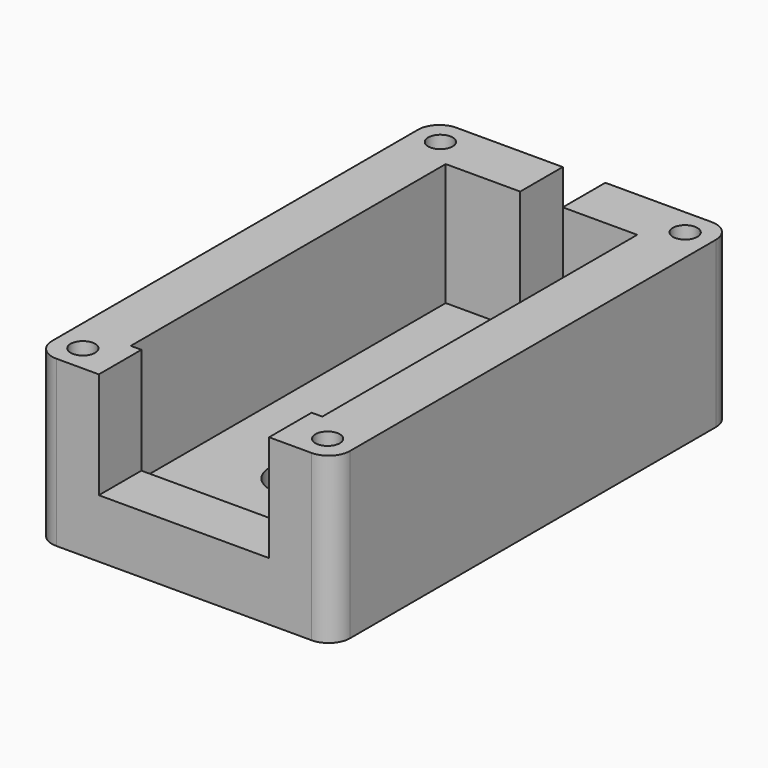
from build123d import *

# Parameters (mm, degrees)
F0_W           = 28
F0_H           = 47
F0_R           = 1.15
F0_W_2         = 18
F0_H_2         = 37
F1_DEPTH       = 11.5
F2_W           = 28
F2_H           = 47
F2_R           = 1.15
F2_W_2         = 18
F2_H_2         = 37
F3_DEPTH       = 4
F4_W           = 16
F4_H           = 5
F4_W_2         = 4
F5_DEPTH       = 10
F6_R           = 2
F8_D           = 2.9
F8_CBORE_D     = 5.5
F8_CBORE_DEPTH = 2.5


with BuildPart() as f1:
    # F0 (on Top) → F1 (new body)
    with BuildSketch(Plane.XY):
        Rectangle(F0_W, F0_H)
        with Locations((-11.5, -21)):
            Circle(F0_R, mode=Mode.SUBTRACT)
        with Locations((11.5, -21)):
            Circle(F0_R, mode=Mode.SUBTRACT)
        with Locations((-11.5, 21)):
            Circle(F0_R, mode=Mode.SUBTRACT)
        Rectangle(F0_W_2, F0_H_2, mode=Mode.SUBTRACT)
        with Locations((11.5, 21)):
            Circle(F0_R, mode=Mode.SUBTRACT)
    extrude(amount=F1_DEPTH)

    # F2 (on face) → F3 (join)
    with BuildSketch(Plane(origin=(0, 0, 0), x_dir=(1, 0, 0), z_dir=(0, 0, -1))):
        Rectangle(F2_W, F2_H)
        with Locations((-11.5, -21)):
            Circle(F2_R, mode=Mode.SUBTRACT)
        with Locations((11.5, -21)):
            Circle(F2_R, mode=Mode.SUBTRACT)
        with Locations((-11.5, 21)):
            Circle(F2_R, mode=Mode.SUBTRACT)
        Rectangle(F2_W_2, F2_H_2, mode=Mode.SUBTRACT)
        with Locations((11.5, 21)):
            Circle(F2_R, mode=Mode.SUBTRACT)
        with Locations((-11.5, 21)):
            Circle(F2_R)
        with Locations((11.5, 21)):
            Circle(F2_R)
        with Locations((-11.5, -21)):
            Circle(F2_R)
        Rectangle(F2_W_2, F2_H_2)
        with Locations((11.5, -21)):
            Circle(F2_R)
    extrude(amount=F3_DEPTH)

    # F4 (on face) → F5 (cut)
    with BuildSketch(Plane.XY.offset(11.5)):
        with Locations((0, -21)):
            Rectangle(F4_W, F4_H)
        with Locations((0, 21)):
            Rectangle(F4_W_2, F4_H)
    extrude(amount=-F5_DEPTH, mode=Mode.SUBTRACT)

    # F6
    f6_edges = [f1.edges().sort_by_distance(p)[0] for p in [
        (-14, 23.5, 3.75),
        (14, 23.5, 3.75),
        (14, -23.5, 3.75),
        (-14, -23.5, 3.75),
    ]]
    fillet(f6_edges, radius=F6_R)

    # F8 (through all)
    with Locations(Plane.XY):
        with Locations((0, 10), (0, -10)):
            CounterBoreHole(F8_D / 2, F8_CBORE_D / 2, F8_CBORE_DEPTH)


solid = f1.part
